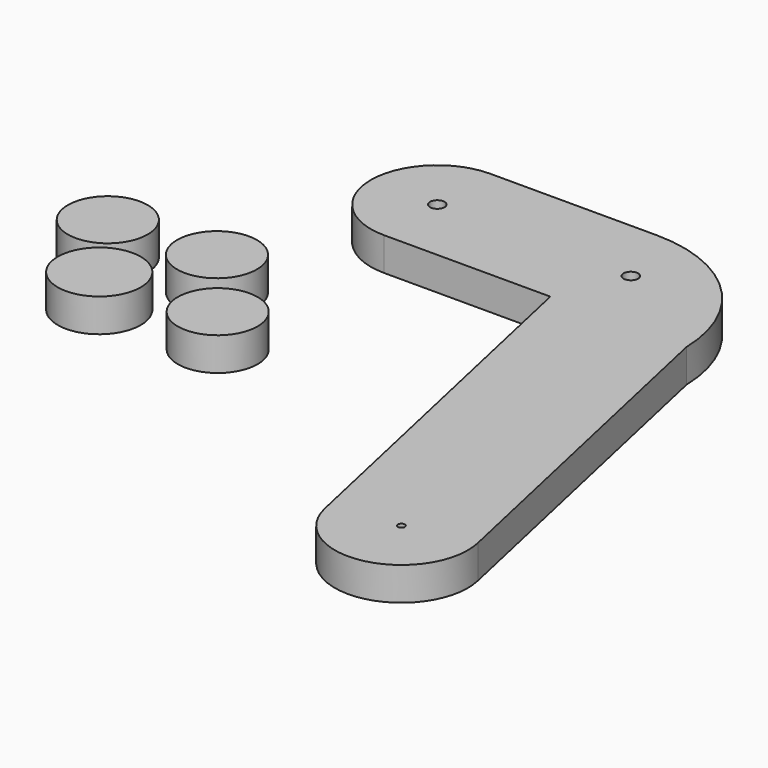
from build123d import *

# Parameters (mm, degrees)
F0_R     = 30.48
F1_DEPTH = 25.4
F0_R_2   = 31.7053585068
F0_R_3   = 2.667
F0_R_4   = 5.5626


# Not quite as in the source:
# - a feature names something its author has since deleted; it is built from what else it names


with BuildPart() as f1:
    # F0 (on Top) → F1 (new body)
    with BuildSketch(Plane.XY):
        with Locations((-209.9951207638, -140.3743773699)):
            Circle(F0_R)
    extrude(amount=F1_DEPTH)


with BuildPart() as f1b:
    # F0 (on Top) → F1, piece 2 (new body)
    with BuildSketch(Plane.XY):
        with Locations((-163.6490523815, -197.625413537)):
            Circle(F0_R)
    extrude(amount=F1_DEPTH)


with BuildPart() as f1c:
    # F0 (on Top) → F1, piece 3 (new body)
    with BuildSketch(Plane.XY):
        with Locations((-250.8887052536, -201.7147690058)):
            Circle(F0_R_2)
    extrude(amount=F1_DEPTH)


with BuildPart() as f1d:
    # F0 (on Top) → F1, piece 4 (new body)
    with BuildSketch(Plane.XY):
        with Locations((-289.0560626984, -145.8268612623)):
            Circle(F0_R)
    extrude(amount=F1_DEPTH)


with BuildPart() as f1e:
    # F0 (on Top) → F1, piece 5 (new body)
    with BuildSketch(Plane.XY):
        with BuildLine():
            Line((-147.8555590361, -58.445237577), (-20.8555590361, -58.445237577))
            Line((-20.8555590361, -58.445237577), (45.0250040162, -356.040249988))
            ThreePointArc((45.0250040162, -356.040249988), (105.6042665934, -394.6593248811), (144.2233414865, -334.0800623039))
            Line((144.2233414865, -334.0800623039), (83.204249457, -58.445237577))
            ThreePointArc((83.204249457, -58.445237577), (51.8613642755, 13.5426289801), (-20.8555590361, 43.154762423))
            Line((-20.8555590361, 43.154762423), (-147.8555590361, 43.154762423))
            ThreePointArc((-147.8555590361, 43.154762423), (-198.6555590361, -7.645237577), (-147.8555590361, -58.445237577))
        make_face()
        with Locations((94.6241727513, -345.0601561459)):
            Circle(F0_R_3, mode=Mode.SUBTRACT)
        with Locations((-147.8555590361, -7.645237577)):
            Circle(F0_R_4, mode=Mode.SUBTRACT)
        with Locations((0, -7.645237577)):
            Circle(F0_R_4, mode=Mode.SUBTRACT)
    extrude(amount=F1_DEPTH)


solid = Compound([f1.part, f1b.part, f1c.part, f1d.part, f1e.part])
